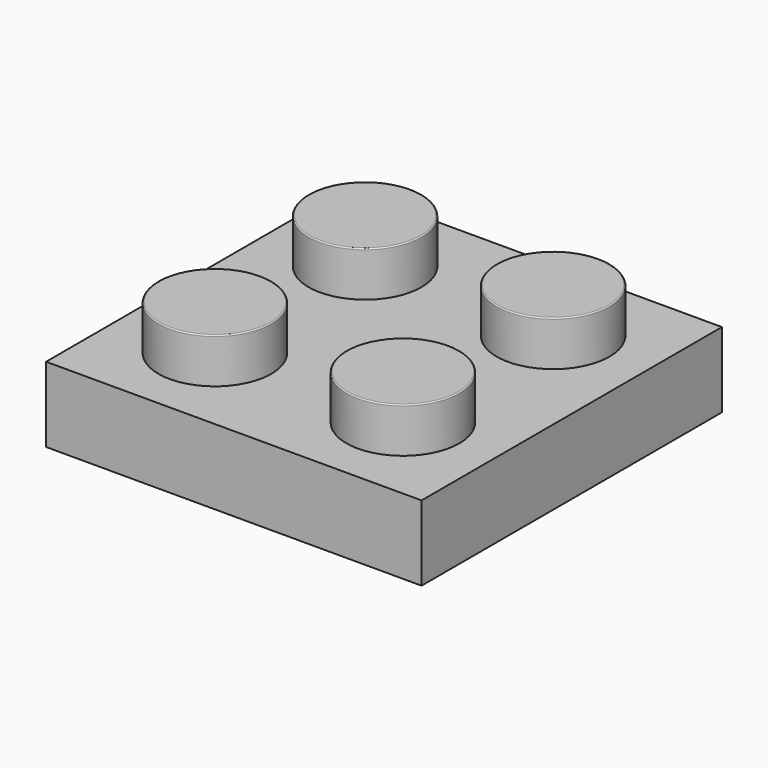
from build123d import *

# Parameters (mm, degrees)
F1_DEPTH = 3.175
F2_DEPTH = 5.08
F3_T     = -1.6002
F4_R     = 0.0508


# Not quite as in the source:
# - a feature names something its author has since deleted; it is built from what else it names


with BuildPart() as f1:
    # F0 (on Top) → F1 (new body)
    with BuildSketch(Plane.XY):
        with BuildLine():
            Line((-22.9340831819, 8.5962191019), (-38.8090831819, 8.5962191019))
            Line((-38.8090831819, 8.5962191019), (-38.8090831819, 4.6274691019))
            Line((-38.8090831819, 4.6274691019), (-37.2342831819, 4.6274691019))
            ThreePointArc((-37.2342831819, 4.6274691019), (-34.8466831819, 7.0150691019), (-32.4590831819, 4.6274691019))
            Line((-32.4590831819, 4.6274691019), (-29.2840831819, 4.6274691019))
            ThreePointArc((-29.2840831819, 4.6274691019), (-26.8964831819, 7.0150691019), (-24.5088831819, 4.6274691019))
            Line((-24.5088831819, 4.6274691019), (-22.9340831819, 4.6274691019))
            Line((-22.9340831819, 4.6274691019), (-22.9340831819, 8.5962191019))
        make_face()
        with BuildLine():
            Line((-37.2342831819, 4.6274691019), (-38.8090831819, 4.6274691019))
            Line((-38.8090831819, 4.6274691019), (-38.8090831819, 0.6587191019))
            Line((-38.8090831819, 0.6587191019), (-22.9340831819, 0.6587191019))
            Line((-22.9340831819, 0.6587191019), (-22.9340831819, 4.6274691019))
            Line((-22.9340831819, 4.6274691019), (-24.5088831819, 4.6274691019))
            ThreePointArc((-24.5088831819, 4.6274691019), (-26.8964831819, 2.2398691019), (-29.2840831819, 4.6274691019))
            Line((-29.2840831819, 4.6274691019), (-32.4590831819, 4.6274691019))
            ThreePointArc((-32.4590831819, 4.6274691019), (-34.8466831819, 2.2398691019), (-37.2342831819, 4.6274691019))
        make_face()
        with BuildLine():
            Line((-37.2342831819, -3.3100308981), (-38.8090831819, -3.3100308981))
            Line((-38.8090831819, -3.3100308981), (-38.8090831819, -7.2787808981))
            Line((-38.8090831819, -7.2787808981), (-22.9340831819, -7.2787808981))
            Line((-22.9340831819, -7.2787808981), (-22.9340831819, -3.3100308981))
            Line((-22.9340831819, -3.3100308981), (-24.5088831819, -3.3100308981))
            ThreePointArc((-24.5088831819, -3.3100308981), (-26.8964831819, -5.6976308981), (-29.2840831819, -3.3100308981))
            Line((-29.2840831819, -3.3100308981), (-32.4590831819, -3.3100308981))
            ThreePointArc((-32.4590831819, -3.3100308981), (-34.8466831819, -5.6976308981), (-37.2342831819, -3.3100308981))
        make_face()
        with BuildLine():
            Line((-22.9340831819, 0.6587191019), (-38.8090831819, 0.6587191019))
            Line((-38.8090831819, 0.6587191019), (-38.8090831819, -3.3100308981))
            Line((-38.8090831819, -3.3100308981), (-37.2342831819, -3.3100308981))
            ThreePointArc((-37.2342831819, -3.3100308981), (-34.8466831819, -0.9224308981), (-32.4590831819, -3.3100308981))
            Line((-32.4590831819, -3.3100308981), (-29.2840831819, -3.3100308981))
            ThreePointArc((-29.2840831819, -3.3100308981), (-26.8964831819, -0.9224308981), (-24.5088831819, -3.3100308981))
            Line((-24.5088831819, -3.3100308981), (-22.9340831819, -3.3100308981))
            Line((-22.9340831819, -3.3100308981), (-22.9340831819, 0.6587191019))
        make_face()
    extrude(amount=F1_DEPTH)

    # F0 (on Top) → F2 (join)
    with BuildSketch(Plane.XY):
        with BuildLine():
            Line((-32.4590831819, 4.6274691019), (-37.2342831819, 4.6274691019))
            ThreePointArc((-37.2342831819, 4.6274691019), (-34.8466831819, 2.2398691019), (-32.4590831819, 4.6274691019))
        make_face()
        with BuildLine():
            ThreePointArc((-32.4590831819, 4.6274691019), (-34.8466831819, 7.0150691019), (-37.2342831819, 4.6274691019))
            Line((-37.2342831819, 4.6274691019), (-32.4590831819, 4.6274691019))
        make_face()
        with BuildLine():
            ThreePointArc((-32.4590831819, -3.3100308981), (-34.8466831819, -0.9224308981), (-37.2342831819, -3.3100308981))
            Line((-37.2342831819, -3.3100308981), (-32.4590831819, -3.3100308981))
        make_face()
        with BuildLine():
            Line((-32.4590831819, -3.3100308981), (-37.2342831819, -3.3100308981))
            ThreePointArc((-37.2342831819, -3.3100308981), (-34.8466831819, -5.6976308981), (-32.4590831819, -3.3100308981))
        make_face()
        with BuildLine():
            ThreePointArc((-29.2840831819, -3.3100308981), (-26.8964831819, -5.6976308981), (-24.5088831819, -3.3100308981))
            Line((-24.5088831819, -3.3100308981), (-29.2840831819, -3.3100308981))
        make_face()
        with BuildLine():
            Line((-29.2840831819, -3.3100308981), (-24.5088831819, -3.3100308981))
            ThreePointArc((-24.5088831819, -3.3100308981), (-26.8964831819, -0.9224308981), (-29.2840831819, -3.3100308981))
        make_face()
        with BuildLine():
            ThreePointArc((-29.2840831819, 4.6274691019), (-26.8964831819, 2.2398691019), (-24.5088831819, 4.6274691019))
            Line((-24.5088831819, 4.6274691019), (-29.2840831819, 4.6274691019))
        make_face()
        with BuildLine():
            Line((-29.2840831819, 4.6274691019), (-24.5088831819, 4.6274691019))
            ThreePointArc((-24.5088831819, 4.6274691019), (-26.8964831819, 7.0150691019), (-29.2840831819, 4.6274691019))
        make_face()
    extrude(amount=F2_DEPTH)

    # F3
    f3_openings = [f1.faces().sort_by_distance(p)[0] for p in [
        (-30.871583, 0.658719, 0),
    ]]
    offset(amount=F3_T, openings=f3_openings, kind=Kind.INTERSECTION)

    # F4
    f4_edges = [f1.edges().sort_by_distance(p)[0] for p in [
        (-32.459083, -3.310031, 5.08),
        (-29.284083, -3.310031, 5.08),
        (-29.284083, 4.627469, 5.08),
        (-37.234283, 4.627469, 5.08),
    ]]
    fillet(f4_edges, radius=F4_R)


solid = f1.part
